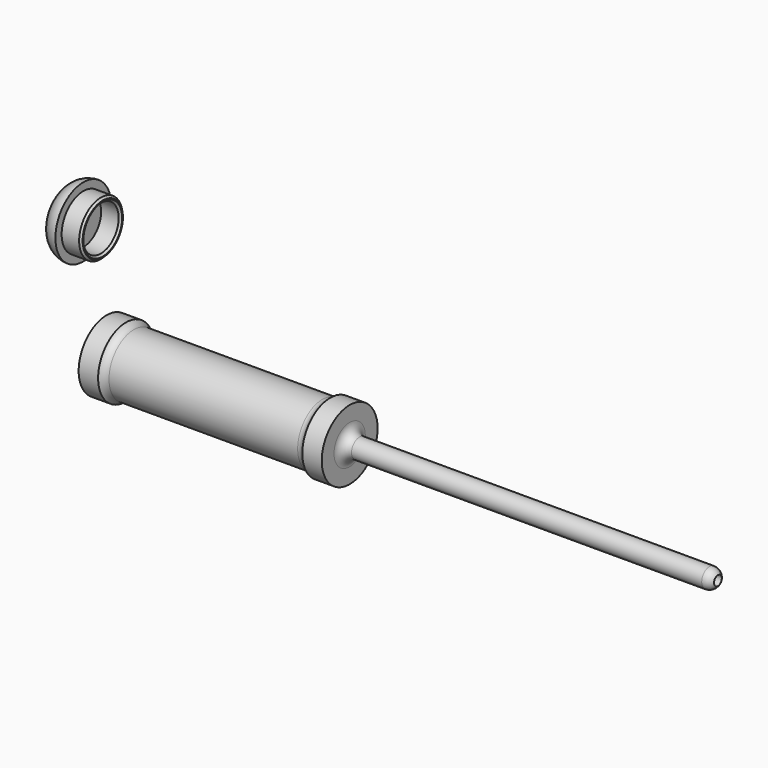
from build123d import *

# Parameters (mm, degrees)
F3_R      = 13.95
F4_DEPTH  = 120
F5_R      = 17.95
F6_DEPTH  = 10
F7_R      = 13.95
F7_R_2    = 11.45
F8_DEPTH  = 10
F9_SIZE   = 1
F10_R     = 9.99999
F11_R     = 2.5
F12_DEPTH = 195.0010001


# Not quite as in the source:
# - a fillet or chamfer that OpenCascade refuses, or shapes differently, is made with other operations: its cross-section is extruded or revolved along the edge and cut away or added
# - a fillet or chamfer is up to 0.001 mm smaller than in the source, because OpenCascade refuses the exact size


with BuildPart() as f1:
    # F0 (on Top) → F1 (revolve)
    with BuildSketch(Plane.XY):
        Polygon((10, 32.9), (0, 32.9), (0, 14.95), (125, 14.95), (315, 14.95), (315, 19.95), (125, 20), (125, 32.9), (115, 32.9), (115, 30.9), (10, 30.9), align=None)
    revolve(axis=Axis((62.5, 14.95, 0), (1, 0, 0)))

    # F2: fillet of radius 5 on 6 edges, made by hand

    # F2_s1 → F2_t2 (revolve)
    with BuildSketch(Plane.XY):
        with BuildLine():
            ThreePointArc((129.9986842106, 19.9986845568), (126.4640009229, 21.4636157101), (125, 24.9986843837))
            Line((125, 24.9986843837), (125, 20))
            Line((125, 20), (129.9986842106, 19.9986845568))
        make_face()
    revolve(axis=Axis((125, 14.95, 0), (1, 0, 0)))

    # F2_s3 → F2_t4 (revolve)
    with BuildSketch(Plane.XY):
        with BuildLine():
            ThreePointArc((111, 30.9), (113.2360679775, 31.427864045), (115, 32.9))
            Line((115, 32.9), (115, 30.9))
            Line((115, 30.9), (111, 30.9))
        make_face()
    revolve(axis=Axis((115, 14.95, 0), (1, 0, 0)))

    # F2_s5 → F2_t6 (revolve)
    with BuildSketch(Plane.XY):
        with BuildLine():
            ThreePointArc((10, 32.9), (11.7639320225, 31.427864045), (14, 30.9))
            Line((14, 30.9), (10, 30.9))
            Line((10, 30.9), (10, 32.9))
        make_face()
    revolve(axis=Axis((10, 14.95, 0), (1, 0, 0)))

    # F2_s7 → F2_t8 (revolve, cut)
    with BuildSketch(Plane.XY):
        with BuildLine():
            ThreePointArc((310.0013157894, 19.9513154432), (313.5359990771, 18.4863842899), (315, 14.9513156163))
            Line((315, 14.9513156163), (315, 19.95))
            Line((315, 19.95), (310.0013157894, 19.9513154432))
        make_face()
    revolve(axis=Axis((315, 14.95, 0), (1, 0, 0)), mode=Mode.SUBTRACT)

    # F3 (on face) → F4 (cut)
    with BuildSketch(Plane(origin=(0, 0, 0), x_dir=(0, -1, 0), z_dir=(-1, 0, 0))):
        with Locations((-14.95, 0)):
            Circle(F3_R)
    extrude(amount=-F4_DEPTH, mode=Mode.SUBTRACT)

    # F11 (on face) → F12 (cut, through all)
    with BuildSketch(Plane(origin=(120, 0, 0), x_dir=(0, -1, 0), z_dir=(-1, 0, 0))):
        with Locations((-14.95, 0)):
            Circle(F11_R)
    extrude(amount=-F12_DEPTH, mode=Mode.SUBTRACT)


with BuildPart() as f6:
    # F5 (on Right) → F6 (new body)
    with BuildSketch(Plane.YZ):
        with Locations((0, 66.2625518771)):
            Circle(F5_R)
    extrude(amount=-F6_DEPTH)

    # F7 (on face) → F8 (join)
    with BuildSketch(Plane.YZ):
        with Locations((0, 66.2625518771)):
            Circle(F7_R)
        with Locations((0, 66.2625518771)):
            Circle(F7_R_2, mode=Mode.SUBTRACT)
    extrude(amount=F8_DEPTH)

    # F9
    f9_edges = [f6.edges().sort_by_distance(p)[0] for p in [
        (10, -13.95, 66.262552),
        (10, -11.45, 66.262552),
    ]]
    chamfer(f9_edges, length=F9_SIZE)

    # F10 (radius 10 in the source; OpenCascade refuses exactly that, so slightly less here)
    f10_edges = [f6.edges().sort_by_distance(p)[0] for p in [
        (-10, -17.95, 66.262552),
    ]]
    fillet(f10_edges, radius=F10_R)


solid = Compound([f1.part, f6.part])
